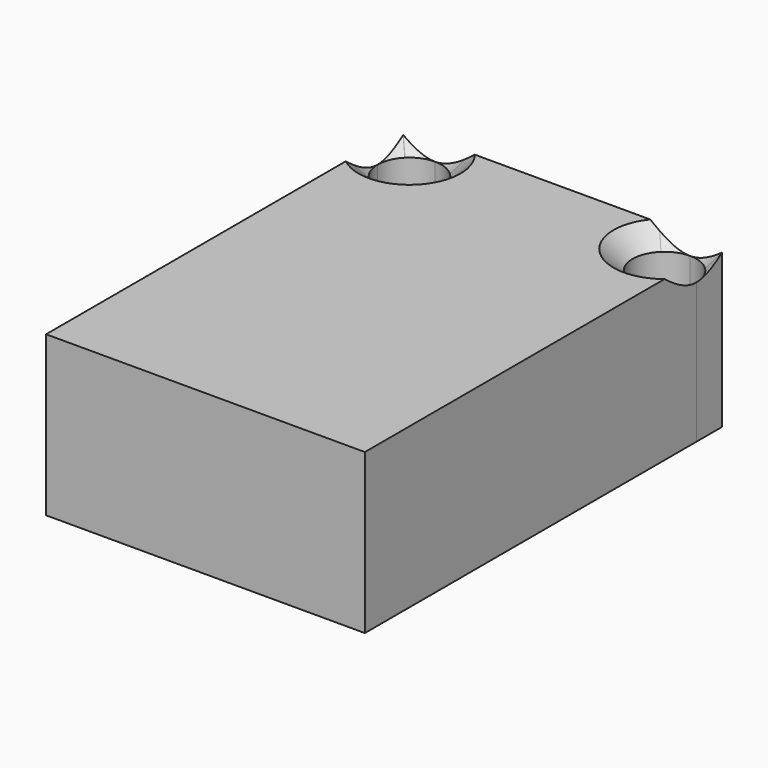
from build123d import *
from build123d import SkipClean  # not in build123d's __all__

# Parameters (mm, degrees)
F1_DEPTH       = 25
F2_DEPTH       = 25.001
F3_T2_ANGLE    = 359.64
F3_T4_ANGLE    = 359.64
F4_T2_ANGLE    = 177.1758988834
F4_S1_T2_ANGLE = 177.1758988834


# Not quite as in the source:
# - a fillet or chamfer that OpenCascade refuses, or shapes differently, is made with other operations: its cross-section is extruded or revolved along the edge and cut away or added


with BuildPart() as f1:
    # F0 (on Top) → F1 (new body)
    with BuildSketch(Plane.XY):
        with BuildLine():
            Line((-20, 35), (-25, 35))
            Line((-25, 35), (-25, 30))
            ThreePointArc((-25, 30), (-23.5355339059, 33.5355339059), (-20, 35))
        make_face()
        with BuildLine():
            Line((19.9999999695, 35), (-20, 35))
            ThreePointArc((-20, 35), (-16.4644660941, 33.5355339059), (-15, 30))
            ThreePointArc((-15, 30), (-20, 25), (-25, 30))
            Line((-25, 30), (-25, -35))
            Line((-25, -35), (25, -35))
            Line((25, -35), (25, 30))
            ThreePointArc((25, 30), (16.4644661049, 26.4644660833), (19.9999999695, 35))
        make_face()
        with BuildLine():
            ThreePointArc((-15, 30), (-16.4644660941, 33.5355339059), (-20, 35))
            ThreePointArc((-20, 35), (-23.5355339059, 33.5355339059), (-25, 30))
            ThreePointArc((-25, 30), (-20, 25), (-15, 30))
        make_face()
        with BuildLine():
            Line((25, 35), (19.9999999695, 35))
            ThreePointArc((19.9999999695, 35), (23.5355338951, 33.5355339167), (25, 30))
            Line((25, 30), (25, 35))
        make_face()
        with BuildLine():
            ThreePointArc((25, 30), (23.5355338951, 33.5355339167), (19.9999999695, 35))
            ThreePointArc((19.9999999695, 35), (16.4644661049, 26.4644660833), (25, 30))
        make_face()
    extrude(amount=F1_DEPTH)

    # F0 (on Top) → F2 (cut, through all)
    with BuildSketch(Plane.XY):
        with BuildLine():
            ThreePointArc((-15, 30), (-16.4644660941, 33.5355339059), (-20, 35))
            ThreePointArc((-20, 35), (-23.5355339059, 33.5355339059), (-25, 30))
            ThreePointArc((-25, 30), (-20, 25), (-15, 30))
        make_face()
        with BuildLine():
            ThreePointArc((25, 30), (23.5355338951, 33.5355339167), (19.9999999695, 35))
            ThreePointArc((19.9999999695, 35), (16.4644661049, 26.4644660833), (25, 30))
        make_face()
    extrude(amount=F2_DEPTH, mode=Mode.SUBTRACT)

    # F3: chamfer of 3 on 2 edges, made by hand

    # F3_s1 → F3_t2 (revolve, cut)
    with BuildSketch(Plane(origin=(-5.062535292, 5.0944444589, 0), x_dir=(0, 0, 1), z_dir=(-0.7048818561, 0.7093247274, 0))):
        Polygon((25, 43.3329502316), (22, 40.3329502316), (25, 40.3329502316), align=None)
    revolve(axis=Axis((20, 30, 25), (0, 0, -1)), revolution_arc=F3_T2_ANGLE, mode=Mode.SUBTRACT)

    # F3_s3 → F3_t4 (revolve, cut)
    with BuildSketch(Plane(origin=(4.9368724732, 4.905950232, 0), x_dir=(0, 0, 1), z_dir=(-0.7093247296, -0.7048818539, 0))):
        Polygon((25, 43.377378966), (22, 40.377378966), (25, 40.377378966), align=None)
    revolve(axis=Axis((-20, 30, 25), (0, 0, -1)), revolution_arc=F3_T4_ANGLE, mode=Mode.SUBTRACT)

    # F4: chamfer of 3 on 1 edges, made by hand

    # F4_s1 → F4_t2 (revolve, cut)
    with BuildSketch(Plane(origin=(-24.4890834382, 25.7269036129, 0), x_dir=(0, 0, 1), z_dir=(0.6894672193, -0.7243168875, 0))):
        Polygon((22, -1.1976788275), (25, 1.8023211725), (25, -1.1976788275), align=None)
    with SkipClean():  # cleaning this boolean's faces spoils the solid; the shape is the same uncleaned
        revolve(axis=Axis((-20, 30, 25), (0, 0, -1)), revolution_arc=F4_T2_ANGLE, mode=Mode.SUBTRACT)

    # F4#s1: chamfer of 3 on 1 edges, made by hand

    # F4_s1_s1 → F4_s1_t2 (revolve, cut)
    with BuildSketch(Plane(origin=(25.4744815239, 24.2488064941, 0), x_dir=(0, 0, 1), z_dir=(-0.7243168854, -0.6894672215, 0))):
        Polygon((22, 12.940162133), (25, 15.940162133), (25, 12.940162133), align=None)
    with SkipClean():  # cleaning this boolean's faces spoils the solid; the shape is the same uncleaned
        revolve(axis=Axis((20, 30, 25), (0, 0, -1)), revolution_arc=F4_S1_T2_ANGLE, mode=Mode.SUBTRACT)


solid = f1.part
